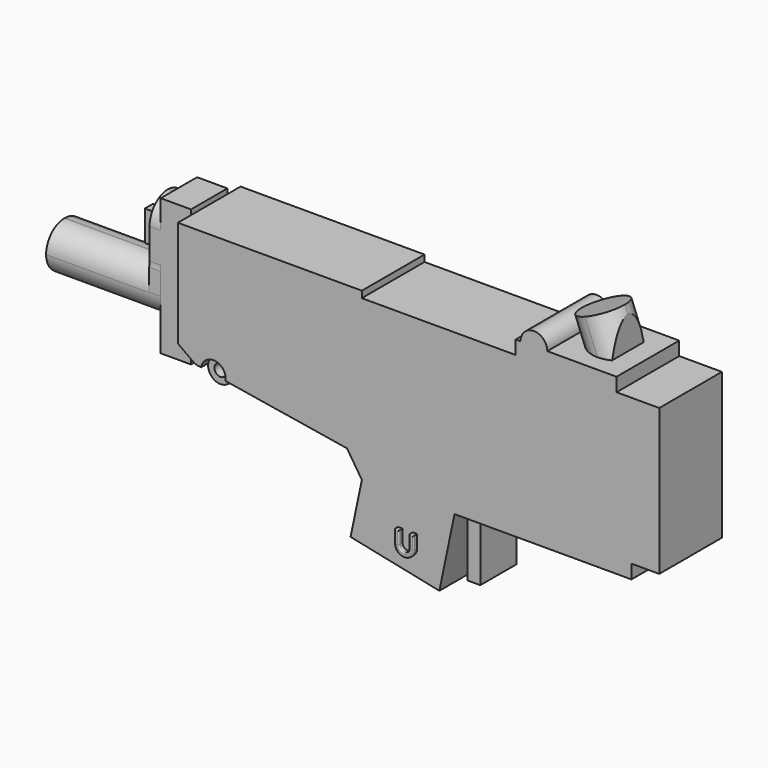
from build123d import *

# Parameters (mm, degrees)
F0_W        = 11
F0_H        = 57.8
F1_DEPTH    = 15.5
F2_DEPTH    = 9.2
F3_DEPTH    = 9
F0_W_2      = 7.5
F0_H_2      = 12
F0_R        = 2.4
F4_DEPTH    = 2
F0_W_3      = 5
F0_H_3      = 25.8
F5_DEPTH    = 9
F6_DEPTH    = 11.95
F7_T4_DEPTH = 55.8672846567
F7_T9_DEPTH = 65.2797771826
F8_T1_DEPTH = 4.4
F8_T3_DEPTH = 27.3945645751
F9_T1_DEPTH = 67.7
F9_T3_DEPTH = 63.3
F12_DEPTH   = 1.8
F13_DEPTH   = 34
F14_R       = 0.5
F15_R       = 0.5


# Not quite as in the source:
# - a fillet or chamfer that OpenCascade refuses, or shapes differently, is made with other operations: its cross-section is extruded or revolved along the edge and cut away or added


with BuildPart() as f1:
    # F0 (on Front) → F1 (new body)
    with BuildSketch(Plane.XZ):
        Polygon((36.6750596455, -31.65), (0, -31.65), (-4.4580704593, -52.9892972654), (30.6832493492, -60.3307986181), align=None)
        with BuildLine():
            Line((0, -31.65), (0, 31.65))
            Line((0, 31.65), (0, 34.25))
            Line((0, 34.25), (-72.8, 34.25))
            Line((-72.8, 34.25), (-72.8, -7.85))
            Line((-72.8, -7.85), (-65.8825243602, -12.7894868936))
            Line((-65.8825243602, -12.7894868936), (-63.6125976921, -13.1602063582))
            ThreePointArc((-63.6125976921, -13.1602063582), (-58.3804729246, -9.066043583), (-53.8766669643, -13.95))
            ThreePointArc((-53.8766669643, -13.95), (-53.8927105474, -14.3461940397), (-53.9407362366, -14.7397936418))
            Line((-53.9407362366, -14.7397936418), (-5.8775063509, -22.5893753474))
            Line((-5.8775063509, -22.5893753474), (0, -31.65))
        make_face()
        Polygon((60.9, 31.65), (0, 31.65), (0, -31.65), (36.6750596455, -31.65), (41.6750596455, -31.65), (106.7, -31.65), (106.7, -26.15), (106.7, 31.65), (100.8, 31.65), align=None)
        with Locations((112.2, 2.75)):
            Rectangle(F0_W, F0_H)
        with BuildLine():
            Line((60.9, 37.05), (60.9, 31.65))
            Line((60.9, 31.65), (100.8, 31.65))
            Line((100.8, 31.65), (100.8, 37.05))
            Line((100.8, 37.05), (92.9, 37.05))
            Line((92.9, 37.05), (78.1969370594, 37.05))
            Line((78.1969370594, 37.05), (73.4, 37.05))
            ThreePointArc((73.4, 37.05), (68.1, 31.75), (62.8, 37.05))
            Line((62.8, 37.05), (60.9, 37.05))
        make_face()
        with BuildLine():
            Line((68.1, 42.35), (68.1, 37.05))
            Line((68.1, 37.05), (73.4, 37.05))
            ThreePointArc((73.4, 37.05), (71.8476659403, 40.7976659403), (68.1, 42.35))
        make_face()
        with BuildLine():
            ThreePointArc((68.1, 42.35), (64.3523340597, 40.7976659403), (62.8, 37.05))
            Line((62.8, 37.05), (68.1, 37.05))
            Line((68.1, 37.05), (68.1, 42.35))
        make_face()
        with BuildLine():
            Line((68.1, 37.05), (62.8, 37.05))
            ThreePointArc((62.8, 37.05), (68.1, 31.75), (73.4, 37.05))
            Line((73.4, 37.05), (68.1, 37.05))
        make_face()
    extrude(amount=F1_DEPTH)



with BuildPart() as f2:
    # F0 (on Front) → F2 (new body)
    with BuildSketch(Plane.XZ):
        Polygon((-130, -6.85), (-84.8, -6.85), (-84.8, 10.95), (-89.2, 10.95), (-130, 10.95), align=None)
    extrude(amount=F2_DEPTH)


with BuildPart() as f1_1:
    add(f1.part)

    add(f2.part)  # F3 merges F2
    # F0 (on Front) → F3 (join)
    with BuildSketch(Plane.XZ):
        Polygon((-72.8, -7.85), (-72.8, 34.25), (-72.8, 36.25), (-84.8, 36.25), (-84.8, 34.25), (-84.8, 10.95), (-84.8, -6.85), (-84.8, -17.7894868936), (-72.8, -17.7894868936), align=None)
        Polygon((-84.8, 10.95), (-84.8, 34.25), (-89.2, 34.25), (-89.2, 25.95), (-89.2, 13.95), (-89.2, 10.95), align=None)
        Polygon((78.1969370594, 37.05), (92.9, 37.05), (92.9, 49.9748528671), (91.7368025022, 52.95), (74.6, 46.25), align=None)
    extrude(amount=F3_DEPTH)

    # F0 (on Front) → F4 (join)
    with BuildSketch(Plane.XZ):
        with Locations((-92.95, 19.95)):
            Rectangle(F0_W_2, F0_H_2)
        with Locations((-92.3, 19.95)):
            Circle(F0_R, mode=Mode.SUBTRACT)
    extrude(amount=F4_DEPTH)

    # F0 (on Front) → F5 (join)
    with BuildSketch(Plane.XZ):
        with Locations((39.1750596455, -44.55)):
            Rectangle(F0_W_3, F0_H_3)
    extrude(amount=F5_DEPTH)

    # F0 (on Front) → F6 (join)
    with BuildSketch(Plane.XZ):
        with BuildLine():
            ThreePointArc((-63.6125976921, -13.1602063582), (-59.5664606062, -18.7859307277), (-53.9407362366, -14.7397936418))
            Line((-53.9407362366, -14.7397936418), (-56.4080478324, -14.3368377021))
            ThreePointArc((-56.4080478324, -14.3368377021), (-59.1635046665, -16.3186191319), (-61.1452860963, -13.5631622979))
            Line((-61.1452860963, -13.5631622979), (-63.6125976921, -13.1602063582))
        make_face()
        with BuildLine():
            Line((-56.4080478324, -14.3368377021), (-53.9407362366, -14.7397936418))
            ThreePointArc((-53.9407362366, -14.7397936418), (-53.8927105474, -14.3461940397), (-53.8766669643, -13.95))
            ThreePointArc((-53.8766669643, -13.95), (-58.3804729246, -9.066043583), (-63.6125976921, -13.1602063582))
            Line((-63.6125976921, -13.1602063582), (-61.1452860963, -13.5631622979))
            ThreePointArc((-61.1452860963, -13.5631622979), (-58.5826127408, -11.5578580815), (-56.3766669643, -13.95))
            ThreePointArc((-56.3766669643, -13.95), (-56.3845250458, -14.1440542235), (-56.4080478324, -14.3368377021))
        make_face()
    extrude(amount=F6_DEPTH)

    # F7: fillet of radius 9.2 on 2 edges, made by hand


with BuildPart() as f7_tool2:
    # F7_s3 → F7_t4 (new body)
    with BuildSketch(Plane(origin=(-14.1665955701, 0, 36.2343508079), x_dir=(0, 1, 0), z_dir=(0.3641304348, 0, -0.9313479621))):
        with BuildLine():
            ThreePointArc((0, 86.3195905796), (-6.3757128891, 89.0831332328), (-9, 95.5174164097))
            Line((-9, 95.5174164097), (-9, 86.3195905796))
            Line((-9, 86.3195905796), (0, 86.3195905796))
        make_face()
    extrude(amount=F7_T4_DEPTH)

    split(bisect_by=Plane.XY.offset(37.05), keep=Keep.TOP)


with BuildPart() as f1_2:
    add(f1_1.part)

    # F7_t1: cut F7_tool2
    add(f7_tool2.part, mode=Mode.SUBTRACT)


with BuildPart() as f7_tool7:
    # F7_s8 → F7_t9 (new body)
    with BuildSketch(Plane(origin=(9.603758078, 0, -24.563836636), x_dir=(0, 1, 0), z_dir=(-0.3641304348, 0, 0.9313479621))):
        with BuildLine():
            ThreePointArc((0, -104.7195905796), (-6.3757128891, -101.9560479264), (-9, -95.5217647496))
            Line((-9, -95.5217647496), (-9, -104.7195905796))
            Line((-9, -104.7195905796), (0, -104.7195905796))
        make_face()
    extrude(amount=F7_T9_DEPTH)

    split(bisect_by=Plane.XY.offset(37.05), keep=Keep.TOP)


with BuildPart() as f1_3:
    add(f1_2.part)

    # F7_t6: cut F7_tool7
    add(f7_tool7.part, mode=Mode.SUBTRACT)

    # F8: fillet of radius 9.2 on 2 edges, made by hand

    # F8_s2 → F8_t1 (join)
    with BuildSketch(Plane.YZ.offset(-89.2)):
        with BuildLine():
            ThreePointArc((-9.2, 10.95), (-9.050136613, 11.8987120982), (-9, 12.8578784028))
            Line((-9, 12.8578784028), (-9, 10.95))
            Line((-9, 10.95), (-9.2, 10.95))
        make_face()
    extrude(amount=F8_T1_DEPTH)

    # F8_s4 → F8_t3 (cut)
    with BuildSketch(Plane.YZ.offset(-112.1945645751)):
        with BuildLine():
            ThreePointArc((0, 34.25), (-6.3757128891, 31.4864573468), (-9, 25.0521741699))
            Line((-9, 25.0521741699), (-9, 34.25))
            Line((-9, 34.25), (0, 34.25))
        make_face()
    extrude(amount=F8_T3_DEPTH, mode=Mode.SUBTRACT)

    # F9: fillet of radius 9 on 2 edges, made by hand

    # F9_s2 → F9_t1 (cut)
    with BuildSketch(Plane.YZ.offset(-152.5)):
        with BuildLine():
            ThreePointArc((-0.2, -6.85), (-6.5639610307, -4.2139610307), (-9.2, 2.15))
            Line((-9.2, 2.15), (-9.2, -6.85))
            Line((-9.2, -6.85), (-0.2, -6.85))
        make_face()
    extrude(amount=F9_T1_DEPTH, mode=Mode.SUBTRACT)

    # F9_s4 → F9_t3 (cut)
    with BuildSketch(Plane.YZ.offset(-152.5)):
        with BuildLine():
            ThreePointArc((-9.2, 1.95), (-6.5639610307, 8.3139610307), (-0.2, 10.95))
            Line((-0.2, 10.95), (-9.2, 10.95))
            Line((-9.2, 10.95), (-9.2, 1.95))
        make_face()
    extrude(amount=F9_T3_DEPTH, mode=Mode.SUBTRACT)

    # F10: F1 across plane


with BuildPart() as f1_4:
    add(f1_3.part)
    add(f1_3.part.mirror(Plane.XZ))

    # F11 (on face) → F12 (join)
    with BuildSketch(Plane.XZ.offset(15.5)):
        with BuildLine():
            ThreePointArc((14.3233330357, -48.3658756971), (14.8036945011, -46.5165514962), (16.1233330357, -45.1347768128))
            Line((16.1233330357, -45.1347768128), (16.1233330357, -43.3658756971))
            Line((16.1233330357, -43.3658756971), (14.3233330357, -43.3658756971))
            Line((14.3233330357, -43.3658756971), (14.3233330357, -48.3658756971))
        make_face()
        with BuildLine():
            Line((18.1233330357, -52.1658756971), (18.1233330357, -50.8158756971))
            ThreePointArc((18.1233330357, -50.8158756971), (15.9473863376, -49.4918223952), (16.1233330357, -46.9507785273))
            Line((16.1233330357, -46.9507785273), (16.1233330357, -45.1347768128))
            ThreePointArc((16.1233330357, -45.1347768128), (14.8036945011, -46.5165514962), (14.3233330357, -48.3658756971))
            ThreePointArc((14.3233330357, -48.3658756971), (15.4363272672, -51.0528814656), (18.1233330357, -52.1658756971))
        make_face()
        with BuildLine():
            ThreePointArc((16.1233330357, -46.9507785273), (15.9473863376, -49.4918223952), (18.1233330357, -50.8158756971))
            Line((18.1233330357, -50.8158756971), (18.1233330357, -50.3658756971))
            ThreePointArc((18.1233330357, -50.3658756971), (16.7091194733, -49.7800892595), (16.1233330357, -48.3658756971))
            Line((16.1233330357, -48.3658756971), (16.1233330357, -46.9507785273))
        make_face()
        with BuildLine():
            ThreePointArc((18.1233330357, -50.8158756971), (19.8557446496, -50.098287311), (20.5733330357, -48.3658756971))
            ThreePointArc((20.5733330357, -48.3658756971), (20.4581242469, -47.6234135769), (20.1233330357, -46.9507785273))
            Line((20.1233330357, -46.9507785273), (20.1233330357, -48.3658756971))
            ThreePointArc((20.1233330357, -48.3658756971), (19.537546598, -49.7800892595), (18.1233330357, -50.3658756971))
            Line((18.1233330357, -50.3658756971), (18.1233330357, -50.8158756971))
        make_face()
        with BuildLine():
            ThreePointArc((20.1233330357, -46.9507785273), (20.4581242469, -47.6234135769), (20.5733330357, -48.3658756971))
            ThreePointArc((20.5733330357, -48.3658756971), (19.8557446496, -50.098287311), (18.1233330357, -50.8158756971))
            Line((18.1233330357, -50.8158756971), (18.1233330357, -52.1658756971))
            ThreePointArc((18.1233330357, -52.1658756971), (20.8103388042, -51.0528814656), (21.9233330357, -48.3658756971))
            ThreePointArc((21.9233330357, -48.3658756971), (21.4429715702, -46.5165514962), (20.1233330357, -45.1347768128))
            Line((20.1233330357, -45.1347768128), (20.1233330357, -46.9507785273))
        make_face()
        with BuildLine():
            Line((20.1233330357, -43.3658756971), (20.1233330357, -45.1347768128))
            ThreePointArc((20.1233330357, -45.1347768128), (21.4429715702, -46.5165514962), (21.9233330357, -48.3658756971))
            Line((21.9233330357, -48.3658756971), (21.9233330357, -43.3658756971))
            Line((21.9233330357, -43.3658756971), (20.1233330357, -43.3658756971))
        make_face()
    extrude(amount=F12_DEPTH)

    # F11 (on face) → F13 (join)
    with BuildSketch(Plane.XZ.offset(15.5)):
        with BuildLine():
            ThreePointArc((16.1233330357, -46.9507785273), (15.9473863376, -49.4918223952), (18.1233330357, -50.8158756971))
            Line((18.1233330357, -50.8158756971), (18.1233330357, -50.3658756971))
            ThreePointArc((18.1233330357, -50.3658756971), (16.7091194733, -49.7800892595), (16.1233330357, -48.3658756971))
            Line((16.1233330357, -48.3658756971), (16.1233330357, -46.9507785273))
        make_face()
        with BuildLine():
            Line((20.1233330357, -48.3658756971), (20.1233330357, -46.9507785273))
            ThreePointArc((20.1233330357, -46.9507785273), (18.1233330357, -45.9158756971), (16.1233330357, -46.9507785273))
            Line((16.1233330357, -46.9507785273), (16.1233330357, -48.3658756971))
            ThreePointArc((16.1233330357, -48.3658756971), (18.1233330357, -46.3658756971), (20.1233330357, -48.3658756971))
        make_face()
        with BuildLine():
            ThreePointArc((18.1233330357, -50.8158756971), (19.8557446496, -50.098287311), (20.5733330357, -48.3658756971))
            ThreePointArc((20.5733330357, -48.3658756971), (20.4581242469, -47.6234135769), (20.1233330357, -46.9507785273))
            Line((20.1233330357, -46.9507785273), (20.1233330357, -48.3658756971))
            ThreePointArc((20.1233330357, -48.3658756971), (19.537546598, -49.7800892595), (18.1233330357, -50.3658756971))
            Line((18.1233330357, -50.3658756971), (18.1233330357, -50.8158756971))
        make_face()
        with BuildLine():
            ThreePointArc((18.1233330357, -50.3658756971), (19.537546598, -49.7800892595), (20.1233330357, -48.3658756971))
            ThreePointArc((20.1233330357, -48.3658756971), (18.1233330357, -46.3658756971), (16.1233330357, -48.3658756971))
            ThreePointArc((16.1233330357, -48.3658756971), (16.7091194733, -49.7800892595), (18.1233330357, -50.3658756971))
        make_face()
    extrude(amount=-F13_DEPTH)

    # F14
    f14_edges = [f1_4.edges().sort_by_distance(p)[0] for p in [
        (18.123333, 18.5, -45.915876),
    ]]
    fillet(f14_edges, radius=F14_R)

    # F15
    f15_edges = [f1_4.edges().sort_by_distance(p)[0] for p in [
        (14.323333, -17.3, -45.865876),
        (18.123333, -17.3, -52.165876),
        (16.123333, -17.3, -45.865876),
        (21.023333, -17.3, -43.365876),
        (15.223333, -17.3, -43.365876),
        (21.923333, -17.3, -45.865876),
        (20.123333, -17.3, -45.865876),
        (18.123333, -17.3, -50.365876),
    ]]
    fillet(f15_edges, radius=F15_R)


solid = f1_4.part
